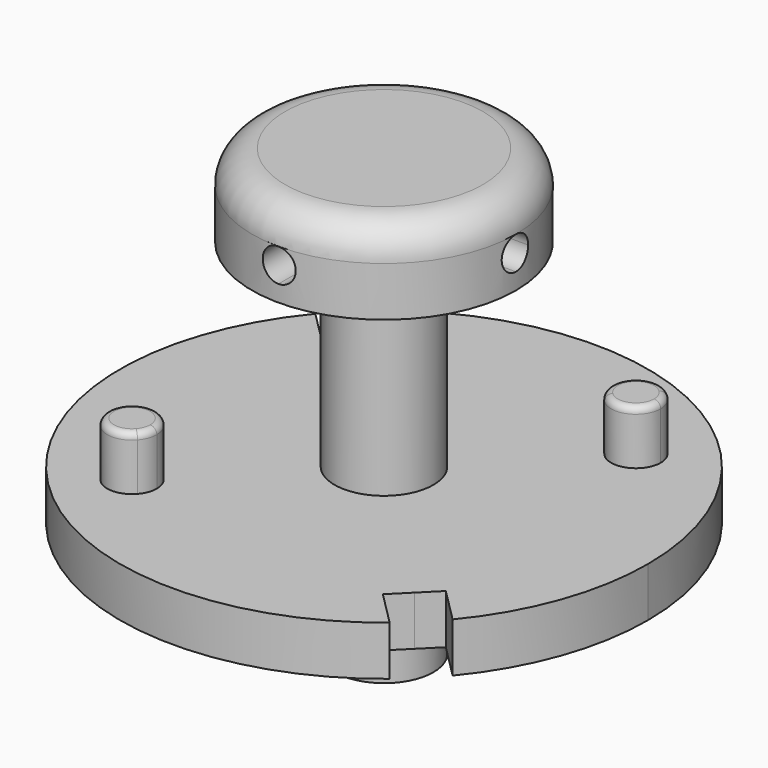
from build123d import *

# Parameters (mm, degrees)
F0_R      = 19.05
F1_DEPTH  = 76.2
F2_R      = 50.8
F2_R_2    = 19.05
F3_DEPTH  = 31.75
F4_R      = 12.7
F7_DEPTH  = 16.002
F10_DEPTH = 16.002
F13_DEPTH = 16.002
F16_DEPTH = 16.002
F18_DEPTH = 19.05
F20_DEPTH = 20.828
F21_R     = 2.54
F22_R     = 25.4
F23_DEPTH = 19.05
F24_R     = 19.05
F25_DEPTH = 25.4


with BuildPart() as f1:
    # F0 (on Top) → F1 (new body)
    with BuildSketch(Plane.XY):
        Circle(F0_R)
    extrude(amount=F1_DEPTH)

    # F2 (on face) → F3 (join)
    with BuildSketch(Plane.XY.offset(76.2)):
        Circle(F2_R)
        Circle(F2_R_2, mode=Mode.SUBTRACT)
        Circle(F2_R_2)
    extrude(amount=F3_DEPTH)

    # F4
    f4_edges = [f1.edges().sort_by_distance(p)[0] for p in [
        (-50.8, 0, 107.95),
    ]]
    fillet(f4_edges, radius=F4_R)

    # F6 (on offset) → F7 (cut)
    with BuildSketch(Plane.XZ.offset(50.8)):
        with BuildLine():
            ThreePointArc((0, 82.55), (4.4901280605, 84.4098719395), (6.35, 88.9))
            ThreePointArc((6.35, 88.9), (-4.4901280605, 93.3901280605), (0, 82.55))
        make_face()
    extrude(amount=-F7_DEPTH, mode=Mode.SUBTRACT)

    # F9 (on offset) → F10 (cut)
    with BuildSketch(Plane.YZ.offset(-50.8)):
        with BuildLine():
            ThreePointArc((0, 82.55), (4.4901280605, 84.4098719395), (6.35, 88.9))
            ThreePointArc((6.35, 88.9), (-4.4901280605, 93.3901280605), (0, 82.55))
        make_face()
    extrude(amount=F10_DEPTH, mode=Mode.SUBTRACT)

    # F12 (on offset) → F13 (cut)
    with BuildSketch(Plane.XZ.offset(-50.8)):
        with BuildLine():
            ThreePointArc((0, 82.55), (4.4901280605, 84.4098719395), (6.35, 88.9))
            ThreePointArc((6.35, 88.9), (-4.4901280605, 93.3901280605), (0, 82.55))
        make_face()
    extrude(amount=F13_DEPTH, mode=Mode.SUBTRACT)

    # F15 (on offset) → F16 (cut)
    with BuildSketch(Plane.YZ.offset(50.8)):
        with BuildLine():
            ThreePointArc((0, 82.55), (4.4901280605, 84.4098719395), (6.35, 88.9))
            ThreePointArc((6.35, 88.9), (-4.4901280605, 93.3901280605), (0, 82.55))
        make_face()
    extrude(amount=-F16_DEPTH, mode=Mode.SUBTRACT)


with BuildPart() as f18:
    # F17 (on face) → F18 (new body)
    with BuildSketch(Plane(origin=(0, 0, 0), x_dir=(1, 0, 0), z_dir=(0, 0, -1))):
        with BuildLine():
            Line((19.05, 0), (101.6, 0))
            ThreePointArc((101.6, 0), (95.5872913823, 34.4329744025), (78.2608321613, 64.7904479797))
            Line((78.2608321613, 64.7904479797), (65.1068568778, 51.6364726961))
            Line((65.1068568778, 51.6364726961), (58.3716647869, 58.3716647869))
            Line((58.3716647869, 58.3716647869), (13.4703841816, 13.4703841816))
            ThreePointArc((13.4703841816, 13.4703841816), (17.5999050943, 7.2901193866), (19.05, 0))
        make_face()
        with BuildLine():
            ThreePointArc((-64.7904479797, -78.2608321613), (43.2426322352, -91.9382116281), (101.6, 0))
            Line((101.6, 0), (19.05, 0))
            ThreePointArc((19.05, 0), (0, -19.05), (-19.05, 0))
            Line((-19.05, 0), (-101.6, 0))
            ThreePointArc((-101.6, 0), (-95.5872913823, -34.4329744025), (-78.2608321613, -64.7904479797))
            Line((-78.2608321613, -64.7904479797), (-65.1068568778, -51.6364726961))
            Line((-65.1068568778, -51.6364726961), (-58.3716647869, -58.3716647869))
            Line((-58.3716647869, -58.3716647869), (-51.6364726961, -65.1068568778))
            Line((-51.6364726961, -65.1068568778), (-64.7904479797, -78.2608321613))
        make_face()
        with BuildLine():
            ThreePointArc((-19.05, 0), (0, -19.05), (19.05, 0))
            Line((19.05, 0), (0, 0))
            Line((0, 0), (-19.05, 0))
        make_face()
        with BuildLine():
            Line((0, 0), (19.05, 0))
            ThreePointArc((19.05, 0), (17.5999050943, 7.2901193866), (13.4703841816, 13.4703841816))
            Line((13.4703841816, 13.4703841816), (0, 0))
        make_face()
        with BuildLine():
            Line((-13.4703841816, 13.4703841816), (0, 0))
            Line((0, 0), (0, 19.05))
            ThreePointArc((0, 19.05), (-7.2901193866, 17.5999050943), (-13.4703841816, 13.4703841816))
        make_face()
        with BuildLine():
            Line((0, 19.05), (0, 0))
            Line((0, 0), (13.4703841816, 13.4703841816))
            ThreePointArc((13.4703841816, 13.4703841816), (7.2901193866, 17.5999050943), (0, 19.05))
        make_face()
        with BuildLine():
            Line((-19.05, 0), (0, 0))
            Line((0, 0), (-13.4703841816, 13.4703841816))
            ThreePointArc((-13.4703841816, 13.4703841816), (-17.5999050943, 7.2901193866), (-19.05, 0))
        make_face()
        with BuildLine():
            ThreePointArc((0, 19.05), (7.2901193866, 17.5999050943), (13.4703841816, 13.4703841816))
            Line((13.4703841816, 13.4703841816), (58.3716647869, 58.3716647869))
            Line((58.3716647869, 58.3716647869), (51.6364726961, 65.1068568778))
            Line((51.6364726961, 65.1068568778), (64.7904479797, 78.2608321613))
            ThreePointArc((64.7904479797, 78.2608321613), (34.4329744025, 95.5872913823), (0, 101.6))
            Line((0, 101.6), (0, 19.05))
        make_face()
        with BuildLine():
            Line((-101.6, 0), (-19.05, 0))
            ThreePointArc((-19.05, 0), (-17.5999050943, 7.2901193866), (-13.4703841816, 13.4703841816))
            Line((-13.4703841816, 13.4703841816), (-71.8420489686, 71.8420489686))
            ThreePointArc((-71.8420489686, 71.8420489686), (-93.8661605031, 38.8806367283), (-101.6, 0))
        make_face()
        with BuildLine():
            ThreePointArc((-13.4703841816, 13.4703841816), (-7.2901193866, 17.5999050943), (0, 19.05))
            Line((0, 19.05), (0, 101.6))
            ThreePointArc((0, 101.6), (-38.8806367283, 93.8661605031), (-71.8420489686, 71.8420489686))
            Line((-71.8420489686, 71.8420489686), (-13.4703841816, 13.4703841816))
        make_face()
    extrude(amount=F18_DEPTH)

    # F19 (on face) → F20 (join)
    with BuildSketch(Plane.XY):
        with BuildLine():
            ThreePointArc((-60.182611768, -46.7385626735), (-53.8815367264, -53.8815367264), (-46.7385626735, -60.182611768))
            ThreePointArc((-46.7385626735, -60.182611768), (-44.9719224572, -57.2496814046), (-44.3565367264, -53.8815367264))
            ThreePointArc((-44.3565367264, -53.8815367264), (-49.9631260008, -45.1998501169), (-60.182611768, -46.7385626735))
        make_face()
        with BuildLine():
            ThreePointArc((-60.182611768, -46.7385626735), (-60.6167288172, -60.6167288172), (-46.7385626735, -60.182611768))
            ThreePointArc((-46.7385626735, -60.182611768), (-53.8815367264, -53.8815367264), (-60.182611768, -46.7385626735))
        make_face()
        with BuildLine():
            Line((53.8815367264, 53.8815367264), (47.1463446356, 47.1463446356))
            ThreePointArc((47.1463446356, 47.1463446356), (53.5837348875, 44.3611932943), (60.182611768, 46.7385626735))
            ThreePointArc((60.182611768, 46.7385626735), (57.1437924233, 50.4086003325), (53.8815367264, 53.8815367264))
        make_face()
        with BuildLine():
            ThreePointArc((46.7385626735, 60.182611768), (44.3611932943, 53.5837348875), (47.1463446356, 47.1463446356))
            Line((47.1463446356, 47.1463446356), (53.8815367264, 53.8815367264))
            ThreePointArc((53.8815367264, 53.8815367264), (50.4086003325, 57.1437924233), (46.7385626735, 60.182611768))
        make_face()
        with BuildLine():
            ThreePointArc((60.6167288172, 60.6167288172), (53.5837348875, 63.4018801585), (46.7385626735, 60.182611768))
            ThreePointArc((46.7385626735, 60.182611768), (50.4086003325, 57.1437924233), (53.8815367264, 53.8815367264))
            Line((53.8815367264, 53.8815367264), (60.6167288172, 60.6167288172))
        make_face()
        with BuildLine():
            ThreePointArc((53.8815367264, 53.8815367264), (57.1437924233, 50.4086003325), (60.182611768, 46.7385626735))
            ThreePointArc((60.182611768, 46.7385626735), (62.5632233359, 49.9631260008), (63.4065367264, 53.8815367264))
            ThreePointArc((63.4065367264, 53.8815367264), (62.6814892736, 57.5265964197), (60.6167288172, 60.6167288172))
            Line((60.6167288172, 60.6167288172), (53.8815367264, 53.8815367264))
        make_face()
    extrude(amount=F20_DEPTH)

    # F21
    f21_edges = [f18.edges().sort_by_distance(p)[0] for p in [
        (47.580462, 61.024511, 20.828),
        (-63.406537, -53.881537, 20.828),
    ]]
    fillet(f21_edges, radius=F21_R)

    # F22 (on face) → F23 (join)
    with BuildSketch(Plane(origin=(0, 0, -19.05), x_dir=(1, 0, 0), z_dir=(0, 0, -1))):
        Circle(F22_R)
    extrude(amount=F23_DEPTH)

    # F24 (on face) → F25 (join)
    with BuildSketch(Plane(origin=(0, 0, -38.1), x_dir=(1, 0, 0), z_dir=(0, 0, -1))):
        Circle(F24_R)
    extrude(amount=F25_DEPTH)


solid = Compound([f1.part, f18.part])
